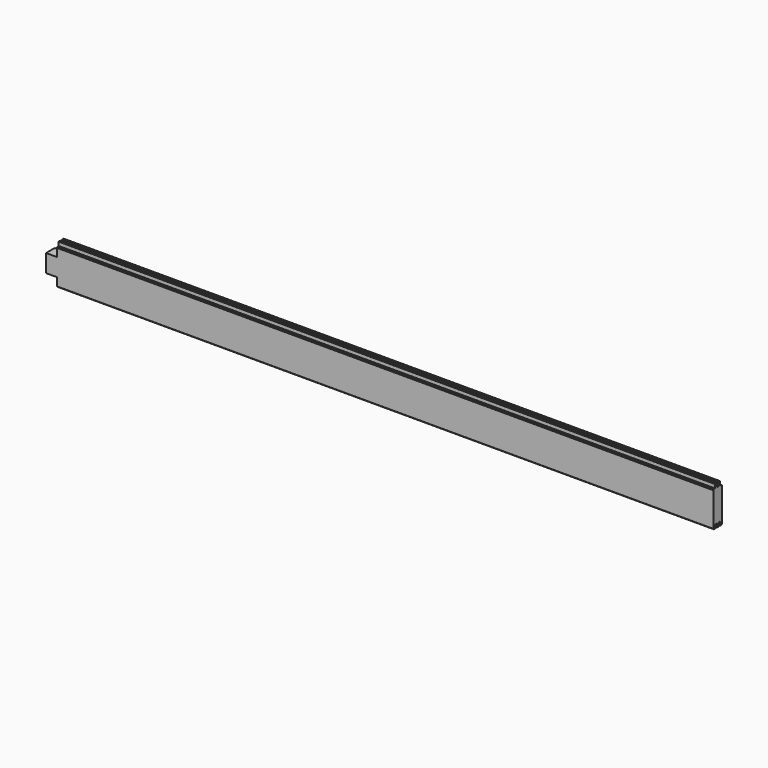
from build123d import *

# Parameters (mm, degrees)
F1_W     = 40
F1_H     = 33
F1_W_2   = 8
F1_H_2   = 14
F3_DEPTH = 1240
F2_W     = 80
F2_H     = 100
F4_DEPTH = 25


with BuildPart() as f3:
    # F1 (on Right) → F3 (new body, symmetric)
    with BuildSketch(Plane.YZ):
        Polygon((20, 33), (20, 63), (17, 66), (12, 66), (12, 80), (4, 80), (4, 66), (-4, 66), (-4, 80), (-12, 80), (-12, 66), (-17, 66), (-20, 63), (-20, 33), align=None)
        with Locations((0, 16.5)):
            Rectangle(F1_W, F1_H)
        with Locations((0, -16.5)):
            Rectangle(F1_W, F1_H)
        Polygon((20, -52), (20, -33), (-20, -33), (-20, -52), (-12, -52), (-4, -52), (4, -52), (12, -52), align=None)
        Polygon((-12, -52), (-20, -52), (-20, -63), (-17, -66), (-12, -66), align=None)
        with Locations((0, -59)):
            Rectangle(F1_W_2, F1_H_2)
        Polygon((20, -63), (20, -52), (12, -52), (12, -66), (17, -66), align=None)
    extrude(amount=F3_DEPTH, both=True)

    # F2 (on Front) → F4 (cut, symmetric)
    with BuildSketch(Plane.XZ):
        with Locations((-1240, 83)):
            Rectangle(F2_W, F2_H)
        with Locations((-1240, -83)):
            Rectangle(F2_W, F2_H)
    extrude(amount=F4_DEPTH, both=True, mode=Mode.SUBTRACT)


solid = f3.part
